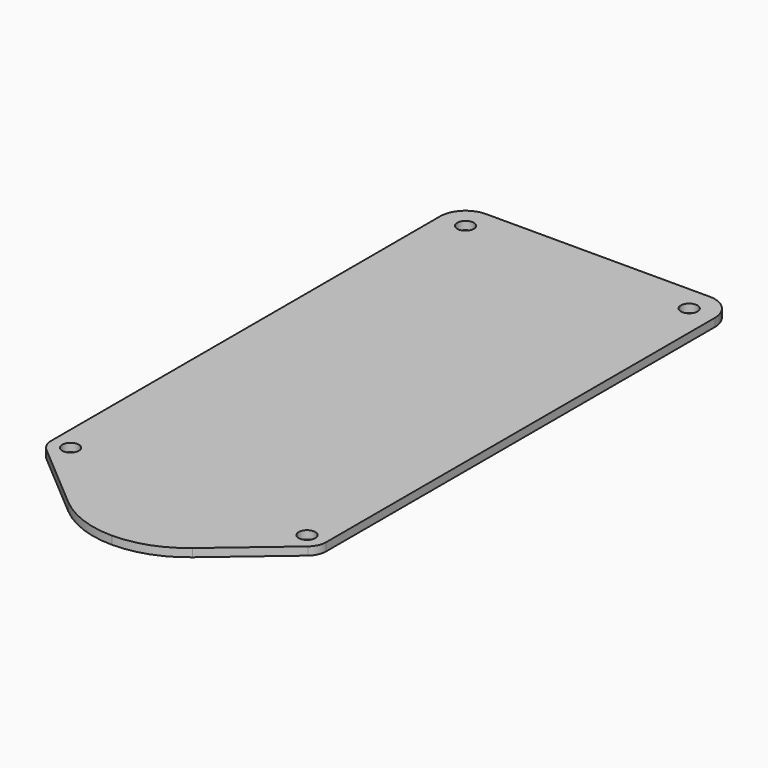
from build123d import *

# Parameters (mm, degrees)
F0_R     = 6.5
F1_DEPTH = 6.35


# Not quite as in the source:
# - a length typed as a fraction of an inch, garbled in the dataset ("3 / 203.2 mm" for 3/8 in), is restored


with BuildPart() as f1:
    # F0 (on Top) → F1 (new body)
    with BuildSketch(Plane.XY):
        with BuildLine():
            Line((0, -75), (0, 0))
            Line((0, 0), (-75, 0))
            ThreePointArc((-75, 0), (-68.0942312118, -31.4352616607), (-48.6486486486, -57.0815993527))
            ThreePointArc((-48.6486486486, -57.0815993527), (-25.9218059609, -70.3779793382), (0, -75))
        make_face()
        with BuildLine():
            ThreePointArc((-48.6486486486, -57.0815993527), (-68.0942312118, -31.4352616607), (-75, 0))
            Line((-75, 0), (-77.5, 0))
            ThreePointArc((-77.5, 0), (-86.2129476679, -13.6188462424), (-102.2297297297, -11.4163198705))
            Line((-102.2297297297, -11.4163198705), (-48.6486486486, -57.0815993527))
        make_face()
        with BuildLine():
            Line((-86, 0), (-77.5, 0))
            ThreePointArc((-77.5, 0), (-86.2129476679, 13.6188462424), (-102.2297297297, 11.4163198705))
            ThreePointArc((-102.2297297297, 11.4163198705), (-106.1188462424, 6.2870523321), (-107.5, 0))
            Line((-107.5, 0), (-99, 0))
            ThreePointArc((-99, 0), (-92.5, 6.5), (-86, 0))
        make_face()
        with BuildLine():
            ThreePointArc((48.6486486486, -57.0815993527), (68.0942312118, -31.4352616607), (75, 0))
            Line((75, 0), (0, 0))
            Line((0, 0), (0, -75))
            ThreePointArc((0, -75), (25.9218059609, -70.3779793382), (48.6486486486, -57.0815993527))
        make_face()
        with BuildLine():
            ThreePointArc((-102.2297297297, -11.4163198705), (-86.2129476679, -13.6188462424), (-77.5, 0))
            Line((-77.5, 0), (-86, 0))
            ThreePointArc((-86, 0), (-92.5, -6.5), (-99, 0))
            Line((-99, 0), (-107.5, 0))
            ThreePointArc((-107.5, 0), (-106.1188462424, -6.2870523321), (-102.2297297297, -11.4163198705))
        make_face()
        with BuildLine():
            ThreePointArc((0, 75), (25.9218059609, 70.3779793382), (48.6486486486, 57.0815993527))
            Line((48.6486486486, 57.0815993527), (102.2297297297, 11.4163198705))
            ThreePointArc((102.2297297297, 11.4163198705), (106.1188462424, 6.2870523321), (107.5, 0))
            Line((107.5, 0), (107.5, 75))
            Line((107.5, 75), (0, 75))
        make_face()
        with BuildLine():
            ThreePointArc((-48.6486486486, 57.0815993527), (-25.9218059609, 70.3779793382), (0, 75))
            Line((0, 75), (107.5, 75))
            Line((107.5, 75), (107.5, 380))
            ThreePointArc((107.5, 380), (101.6421356237, 394.1421356237), (87.5, 400))
            Line((87.5, 400), (-87.5, 400))
            ThreePointArc((-87.5, 400), (-101.6421356237, 394.1421356237), (-107.5, 380))
            Line((-107.5, 380), (-107.5, 0))
            ThreePointArc((-107.5, 0), (-106.1188462424, 6.2870523321), (-102.2297297297, 11.4163198705))
            Line((-102.2297297297, 11.4163198705), (-48.6486486486, 57.0815993527))
        make_face()
        with Locations((-87.5, 380)):
            Circle(F0_R, mode=Mode.SUBTRACT)
        with Locations((87.5, 380)):
            Circle(F0_R, mode=Mode.SUBTRACT)
        with BuildLine():
            Line((86, 0), (77.5, 0))
            ThreePointArc((77.5, 0), (86.2129476679, -13.6188462424), (102.2297297297, -11.4163198705))
            ThreePointArc((102.2297297297, -11.4163198705), (106.1188462424, -6.2870523321), (107.5, 0))
            Line((107.5, 0), (99, 0))
            ThreePointArc((99, 0), (92.5, -6.5), (86, 0))
        make_face()
        with BuildLine():
            ThreePointArc((102.2297297297, 11.4163198705), (86.2129476679, 13.6188462424), (77.5, 0))
            Line((77.5, 0), (86, 0))
            ThreePointArc((86, 0), (92.5, 6.5), (99, 0))
            Line((99, 0), (107.5, 0))
            ThreePointArc((107.5, 0), (106.1188462424, 6.2870523321), (102.2297297297, 11.4163198705))
        make_face()
        with BuildLine():
            ThreePointArc((48.6486486486, 57.0815993527), (68.0942312118, 31.4352616607), (75, 0))
            Line((75, 0), (77.5, 0))
            ThreePointArc((77.5, 0), (86.2129476679, 13.6188462424), (102.2297297297, 11.4163198705))
            Line((102.2297297297, 11.4163198705), (48.6486486486, 57.0815993527))
        make_face()
        with BuildLine():
            Line((77.5, 0), (75, 0))
            ThreePointArc((75, 0), (68.0942312118, -31.4352616607), (48.6486486486, -57.0815993527))
            Line((48.6486486486, -57.0815993527), (102.2297297297, -11.4163198705))
            ThreePointArc((102.2297297297, -11.4163198705), (86.2129476679, -13.6188462424), (77.5, 0))
        make_face()
        with BuildLine():
            Line((0, 0), (75, 0))
            ThreePointArc((75, 0), (68.0942312118, 31.4352616607), (48.6486486486, 57.0815993527))
            ThreePointArc((48.6486486486, 57.0815993527), (25.9218059609, 70.3779793382), (0, 75))
            Line((0, 75), (0, 0))
        make_face()
        with BuildLine():
            Line((-77.5, 0), (-75, 0))
            ThreePointArc((-75, 0), (-68.0942312118, 31.4352616607), (-48.6486486486, 57.0815993527))
            Line((-48.6486486486, 57.0815993527), (-102.2297297297, 11.4163198705))
            ThreePointArc((-102.2297297297, 11.4163198705), (-86.2129476679, 13.6188462424), (-77.5, 0))
        make_face()
        with BuildLine():
            Line((-75, 0), (0, 0))
            Line((0, 0), (0, 75))
            ThreePointArc((0, 75), (-25.9218059609, 70.3779793382), (-48.6486486486, 57.0815993527))
            ThreePointArc((-48.6486486486, 57.0815993527), (-68.0942312118, 31.4352616607), (-75, 0))
        make_face()
    extrude(amount=F1_DEPTH)


solid = f1.part
